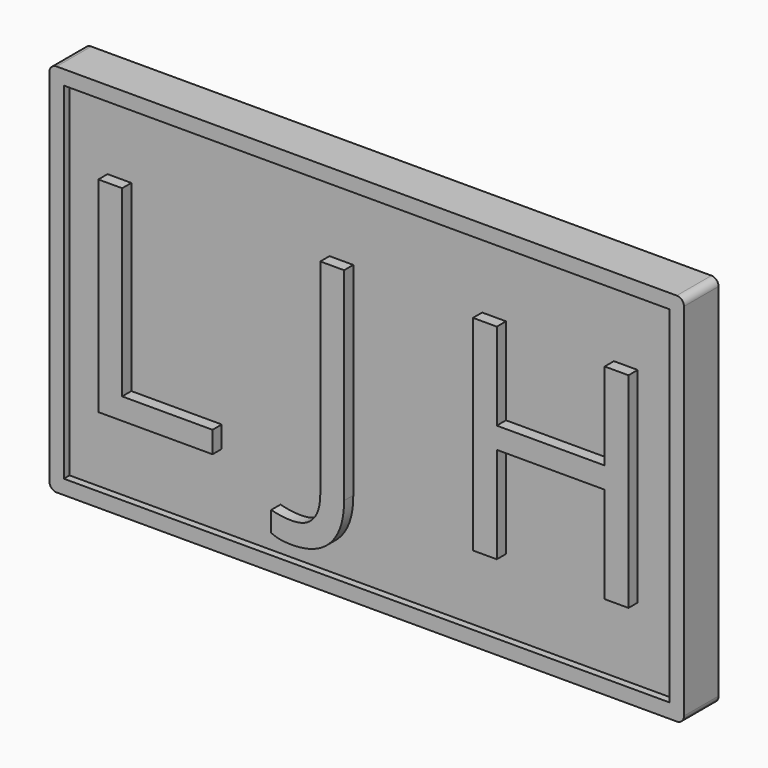
from build123d import *

# Parameters (mm, degrees)
F0_W         = 440
F0_H         = 260
F1_DEPTH     = 30
F2_R         = 5
F3_W         = 420
F3_H         = 240
F4_DEPTH     = 5
F5_R         = 14
F6_DEPTH     = 60
F7_TEXT_SIZE = 198.9276556065
F8_DEPTH     = 33


# Not quite as in the source:
# - a feature of the source that left no trace in its solid (it failed there, or was rolled back) is left out
# - a feature names something its author has since deleted; it is built from what else it names
# - Text() gives the source's letters only with a copy of the font that has no kerning and outlines rounded to 1/6400 em; it was checked with that copy


with BuildPart() as f1:
    # F0 (on Front) → F1 (new body)
    with BuildSketch(Plane.XZ):
        with Locations((150, -90)):
            Rectangle(F0_W, F0_H)
    extrude(amount=F1_DEPTH)

    # F2
    f2_edges = [f1.edges().sort_by_distance(p)[0] for p in [
        (-70, -15, 40),
        (-70, -15, -220),
        (370, -15, 40),
        (370, -15, -220),
    ]]
    fillet(f2_edges, radius=F2_R)

    # F3 (on face) → F4 (cut)
    with BuildSketch(Plane.XZ.offset(30)):
        with Locations((150, -90)):
            Rectangle(F3_W, F3_H)
    extrude(amount=-F4_DEPTH, mode=Mode.SUBTRACT)

    # F5 (on face) → F6 (join)
    with BuildSketch(Plane(origin=(0, 0, 0), x_dir=(-1, 0, 0), z_dir=(0, 1, 0))):
        with Locations((-150, -90)):
            Circle(F5_R)
    extrude(amount=F6_DEPTH)

    # F7 (on Front) → F8 (join)
    with BuildSketch(Plane.XZ):
        with Locations((-53.1886544659, -159.5687167584)):
            Text('L J H', F7_TEXT_SIZE, font='Open Sans', text_align=(TextAlign.LEFT, TextAlign.BOTTOM))
    extrude(amount=F8_DEPTH)


solid = f1.part
